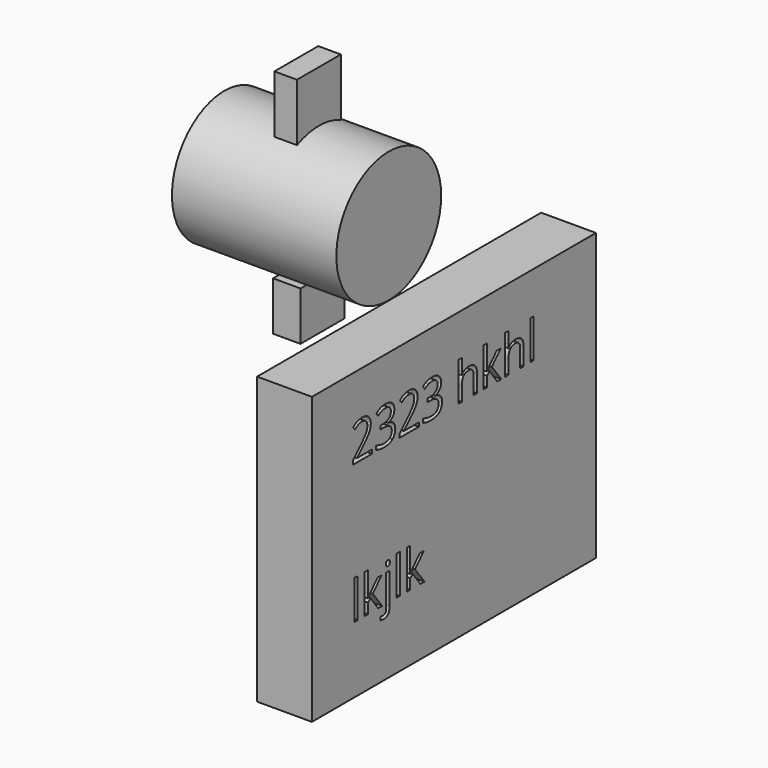
from build123d import *

# Parameters (mm, degrees)
F0_R     = 30.3617666471
F1_DEPTH = 38.1
F2_W     = 12.7535671927
F2_H     = 22.6146032107
F3_DEPTH = 12.7
F4_W     = 10.4644712992
F4_H     = 34.9905658513
F5_DEPTH = 12.7
F6_W     = 164.5638719201
F6_H     = 132.6431203634
F6_W_2   = 1.9235427446
F6_H_2   = 18.0234843295
F7_DEPTH = 25.4


with BuildPart() as f1:
    # F0 (on Right) → F1 (new body, symmetric)
    with BuildSketch(Plane.YZ):
        Circle(F0_R)
    extrude(amount=F1_DEPTH, both=True)

    # F2 (on Front) → F3 (join, symmetric)
    with BuildSketch(Plane.XZ):
        with Locations((0.9810503107, -41.6690682524)):
            Rectangle(F2_W, F2_H)
    extrude(amount=F3_DEPTH, both=True)

    # F4 (on Front) → F5 (join, symmetric)
    with BuildSketch(Plane.XZ):
        with Locations((0.4905241076, 36.7891443893)):
            Rectangle(F4_W, F4_H)
    extrude(amount=F5_DEPTH, both=True)


with BuildPart() as f7:
    # F6 (on face) → F7 (new body)
    with BuildSketch(Plane.YZ.offset(38.1)):
        with Locations((6.0101114213, -96.8088572845)):
            Rectangle(F6_W, F6_H)
        with Locations((-50.736682856, -123.3850151864)):
            Rectangle(F6_W_2, F6_H_2, mode=Mode.SUBTRACT)
        with BuildLine():
            Line((-43.88938956, -125.899704497), (-43.7967333584, -125.899704497))
            add(Edge.make_bspline(
                [(-43.7967333584, -125.899704497), (-43.300096118, -125.191811117), (-42.2808779007, -124.0465804656)],
                knots=[0, 0, 0, 1, 1, 1], degree=2))
            Line((-42.2808779007, -124.0465804656), (-38.1817675432, -119.702857736))
            Line((-38.1817675432, -119.702857736), (-35.8987187365, -119.702857736))
            Line((-35.8987187365, -119.702857736), (-41.0429910477, -125.1102736596))
            Line((-41.0429910477, -125.1102736596), (-35.5392126744, -132.3967573511))
            Line((-35.5392126744, -132.3967573511), (-37.8667364579, -132.3967573511))
            Line((-37.8667364579, -132.3967573511), (-42.3512966139, -126.3963417374))
            Line((-42.3512966139, -126.3963417374), (-43.7967333584, -127.6490535827))
            Line((-43.7967333584, -127.6490535827), (-43.7967333584, -132.3967573511))
            Line((-43.7967333584, -132.3967573511), (-45.6980386146, -132.3967573511))
            Line((-45.6980386146, -132.3967573511), (-45.6980386146, -114.3732730216))
            Line((-45.6980386146, -114.3732730216), (-43.7967333584, -114.3732730216))
            Line((-43.7967333584, -114.3732730216), (-43.7967333584, -123.9316867756))
            add(Edge.make_bspline(
                [(-43.7967333584, -123.9316867756), (-43.7967333584, -124.5654551944), (-43.88938956, -125.899704497)],
                knots=[0, 0, 0, 1, 1, 1], degree=2))
        make_face(mode=Mode.SUBTRACT)
        with BuildLine():
            add(Edge.make_bspline(
                [(-31.325208627, -134.3425375841), (-31.325208627, -138.0969668718), (-34.7905505657, -138.0969668718)],
                knots=[0, 0, 0, 1, 1, 1], degree=2))
            add(Edge.make_bspline(
                [(-34.7905505657, -138.0969668718), (-35.8913062404, -138.0969668718), (-36.5732558839, -137.8041732748)],
                knots=[0, 0, 0, 1, 1, 1], degree=2))
            Line((-36.5732558839, -137.8041732748), (-36.5732558839, -136.2438428403))
            add(Edge.make_bspline(
                [(-36.5732558839, -136.2438428403), (-35.7727063024, -136.4736302202), (-34.9981004572, -136.4736302202)],
                knots=[0, 0, 0, 1, 1, 1], degree=2))
            add(Edge.make_bspline(
                [(-34.9981004572, -136.4736302202), (-34.0937759299, -136.4736302202), (-33.6712636508, -135.9806992279)],
                knots=[0, 0, 0, 1, 1, 1], degree=2))
            add(Edge.make_bspline(
                [(-33.6712636508, -135.9806992279), (-33.2487513716, -135.4877682355), (-33.2487513716, -134.4833750105)],
                knots=[0, 0, 0, 1, 1, 1], degree=2))
            Line((-33.2487513716, -134.4833750105), (-33.2487513716, -119.702857736))
            Line((-33.2487513716, -119.702857736), (-31.325208627, -119.702857736))
            Line((-31.325208627, -119.702857736), (-31.325208627, -134.3425375841))
        make_face(mode=Mode.SUBTRACT)
        with Locations((-26.2865643856, -123.3850151864)):
            Rectangle(F6_W_2, F6_H_2, mode=Mode.SUBTRACT)
        with BuildLine():
            Line((-19.4392710895, -125.899704497), (-19.3466148879, -125.899704497))
            add(Edge.make_bspline(
                [(-19.3466148879, -125.899704497), (-18.8499776475, -125.191811117), (-17.8307594302, -124.0465804656)],
                knots=[0, 0, 0, 1, 1, 1], degree=2))
            Line((-17.8307594302, -124.0465804656), (-13.7316490728, -119.702857736))
            Line((-13.7316490728, -119.702857736), (-11.4486002661, -119.702857736))
            Line((-11.4486002661, -119.702857736), (-16.5928725773, -125.1102736596))
            Line((-16.5928725773, -125.1102736596), (-11.089094204, -132.3967573511))
            Line((-11.089094204, -132.3967573511), (-13.4166179874, -132.3967573511))
            Line((-13.4166179874, -132.3967573511), (-17.9011781434, -126.3963417374))
            Line((-17.9011781434, -126.3963417374), (-19.3466148879, -127.6490535827))
            Line((-19.3466148879, -127.6490535827), (-19.3466148879, -132.3967573511))
            Line((-19.3466148879, -132.3967573511), (-21.2479201442, -132.3967573511))
            Line((-21.2479201442, -132.3967573511), (-21.2479201442, -114.3732730216))
            Line((-21.2479201442, -114.3732730216), (-19.3466148879, -114.3732730216))
            Line((-19.3466148879, -114.3732730216), (-19.3466148879, -123.9316867756))
            add(Edge.make_bspline(
                [(-19.3466148879, -123.9316867756), (-19.3466148879, -124.5654551944), (-19.4392710895, -125.899704497)],
                knots=[0, 0, 0, 1, 1, 1], degree=2))
        make_face(mode=Mode.SUBTRACT)
        with BuildLine():
            add(Edge.make_bspline(
                [(-33.0875295809, -117.2307902781), (-33.4118262864, -116.9120529447), (-33.4118262864, -116.2634595337)],
                knots=[0, 0, 0, 1, 1, 1], degree=2))
            add(Edge.make_bspline(
                [(-33.4118262864, -116.2634595337), (-33.4118262864, -115.6037473785), (-33.0875295809, -115.2961287893)],
                knots=[0, 0, 0, 1, 1, 1], degree=2))
            add(Edge.make_bspline(
                [(-33.0875295809, -115.2961287893), (-32.7632328754, -114.9885102), (-32.2740081311, -114.9885102)],
                knots=[0, 0, 0, 1, 1, 1], degree=2))
            add(Edge.make_bspline(
                [(-32.2740081311, -114.9885102), (-31.8107271232, -114.9885102), (-31.4753116735, -115.3016881614)],
                knots=[0, 0, 0, 1, 1, 1], degree=2))
            add(Edge.make_bspline(
                [(-31.4753116735, -115.3016881614), (-31.1398962238, -115.6148661227), (-31.1398962238, -116.2634595337)],
                knots=[0, 0, 0, 1, 1, 1], degree=2))
            add(Edge.make_bspline(
                [(-31.1398962238, -116.2634595337), (-31.1398962238, -116.9120529447), (-31.4753116735, -117.2307902781)],
                knots=[0, 0, 0, 1, 1, 1], degree=2))
            add(Edge.make_bspline(
                [(-31.4753116735, -117.2307902781), (-31.8107271232, -117.5495276115), (-32.2740081311, -117.5495276115)],
                knots=[0, 0, 0, 1, 1, 1], degree=2))
            add(Edge.make_bspline(
                [(-32.2740081311, -117.5495276115), (-32.7632328754, -117.5495276115), (-33.0875295809, -117.2307902781)],
                knots=[0, 0, 0, 1, 1, 1], degree=2))
        make_face(mode=Mode.SUBTRACT)
        with BuildLine():
            Line((-41.4469720866, -66.0956857553), (-41.4469720866, -67.8783910735))
            Line((-41.4469720866, -67.8783910735), (-52.5768350192, -67.8783910735))
            Line((-52.5768350192, -67.8783910735), (-52.5768350192, -66.2216981894))
            Line((-52.5768350192, -66.2216981894), (-48.1182185996, -61.7408442815))
            add(Edge.make_bspline(
                [(-48.1182185996, -61.7408442815), (-46.0797821651, -59.6764641105), (-45.4311887541, -58.7962301955)],
                knots=[0, 0, 0, 1, 1, 1], degree=2))
            add(Edge.make_bspline(
                [(-45.4311887541, -58.7962301955), (-44.7825953431, -57.9159962806), (-44.4582986376, -57.0820904665)],
                knots=[0, 0, 0, 1, 1, 1], degree=2))
            add(Edge.make_bspline(
                [(-44.4582986376, -57.0820904665), (-44.1340019321, -56.2481846524), (-44.1340019321, -55.2882664041)],
                knots=[0, 0, 0, 1, 1, 1], degree=2))
            add(Edge.make_bspline(
                [(-44.1340019321, -55.2882664041), (-44.1340019321, -53.9317796131), (-44.9567890021, -53.1386425276)],
                knots=[0, 0, 0, 1, 1, 1], degree=2))
            add(Edge.make_bspline(
                [(-44.9567890021, -53.1386425276), (-45.779576072, -52.3455054422), (-47.2398378088, -52.3455054422)],
                knots=[0, 0, 0, 1, 1, 1], degree=2))
            add(Edge.make_bspline(
                [(-47.2398378088, -52.3455054422), (-48.2924122586, -52.3455054422), (-49.2375055146, -52.6938927601)],
                knots=[0, 0, 0, 1, 1, 1], degree=2))
            add(Edge.make_bspline(
                [(-49.2375055146, -52.6938927601), (-50.1825987706, -53.042280078), (-51.3389481662, -53.9577233495)],
                knots=[0, 0, 0, 1, 1, 1], degree=2))
            Line((-51.3389481662, -53.9577233495), (-52.3581663835, -52.6494177833))
            add(Edge.make_bspline(
                [(-52.3581663835, -52.6494177833), (-50.0195238559, -50.7036375504), (-47.2620752971, -50.7036375504)],
                knots=[0, 0, 0, 1, 1, 1], degree=2))
            add(Edge.make_bspline(
                [(-47.2620752971, -50.7036375504), (-44.8752515447, -50.7036375504), (-43.5206178777, -51.9248462871)],
                knots=[0, 0, 0, 1, 1, 1], degree=2))
            add(Edge.make_bspline(
                [(-43.5206178777, -51.9248462871), (-42.1659842107, -53.1460550238), (-42.1659842107, -55.2067289467)],
                knots=[0, 0, 0, 1, 1, 1], degree=2))
            add(Edge.make_bspline(
                [(-42.1659842107, -55.2067289467), (-42.1659842107, -56.818946854), (-43.0703087381, -58.3941022807)],
                knots=[0, 0, 0, 1, 1, 1], degree=2))
            add(Edge.make_bspline(
                [(-43.0703087381, -58.3941022807), (-43.9746332654, -59.9692577074), (-46.4504069714, -62.3783189483)],
                knots=[0, 0, 0, 1, 1, 1], degree=2))
            Line((-46.4504069714, -62.3783189483), (-50.1566550342, -66.0030295537))
            Line((-50.1566550342, -66.0030295537), (-50.1566550342, -66.0956857553))
            Line((-50.1566550342, -66.0956857553), (-41.4469720866, -66.0956857553))
        make_face(mode=Mode.SUBTRACT)
        with BuildLine():
            add(Edge.make_bspline(
                [(-29.8908906267, -51.8321900855), (-28.5232850915, -52.9607426206), (-28.5232850915, -54.928760342)],
                knots=[0, 0, 0, 1, 1, 1], degree=2))
            add(Edge.make_bspline(
                [(-28.5232850915, -54.928760342), (-28.5232850915, -56.5520969935), (-29.4331689909, -57.582433955)],
                knots=[0, 0, 0, 1, 1, 1], degree=2))
            add(Edge.make_bspline(
                [(-29.4331689909, -57.582433955), (-30.3430528903, -58.6127709164), (-32.0108645186, -58.9611582343)],
                knots=[0, 0, 0, 1, 1, 1], degree=2))
            Line((-32.0108645186, -58.9611582343), (-32.0108645186, -59.0538144359))
            add(Edge.make_bspline(
                [(-32.0108645186, -59.0538144359), (-29.9724280841, -59.3058393042), (-28.9884192234, -60.3491481339)],
                knots=[0, 0, 0, 1, 1, 1], degree=2))
            add(Edge.make_bspline(
                [(-28.9884192234, -60.3491481339), (-28.0044103627, -61.3924569636), (-28.0044103627, -63.0825060802)],
                knots=[0, 0, 0, 1, 1, 1], degree=2))
            add(Edge.make_bspline(
                [(-28.0044103627, -63.0825060802), (-28.0044103627, -65.5026860652), (-29.6833407352, -66.8072853833)],
                knots=[0, 0, 0, 1, 1, 1], degree=2))
            add(Edge.make_bspline(
                [(-29.6833407352, -66.8072853833), (-31.3622711076, -68.1118847015), (-34.453281992, -68.1118847015)],
                knots=[0, 0, 0, 1, 1, 1], degree=2))
            add(Edge.make_bspline(
                [(-34.453281992, -68.1118847015), (-35.7986500388, -68.1118847015), (-36.9160838298, -67.908041058)],
                knots=[0, 0, 0, 1, 1, 1], degree=2))
            add(Edge.make_bspline(
                [(-36.9160838298, -67.908041058), (-38.0335176207, -67.7041974145), (-39.0860920705, -67.1964414299)],
                knots=[0, 0, 0, 1, 1, 1], degree=2))
            Line((-39.0860920705, -67.1964414299), (-39.0860920705, -65.3655548869))
            add(Edge.make_bspline(
                [(-39.0860920705, -65.3655548869), (-37.9853363959, -65.9103733521), (-36.7400370468, -66.1939013289)],
                knots=[0, 0, 0, 1, 1, 1], degree=2))
            add(Edge.make_bspline(
                [(-36.7400370468, -66.1939013289), (-35.4947376977, -66.4774293057), (-34.3828632788, -66.4774293057)],
                knots=[0, 0, 0, 1, 1, 1], degree=2))
            add(Edge.make_bspline(
                [(-34.3828632788, -66.4774293057), (-29.9946655724, -66.4774293057), (-29.9946655724, -63.0380311034)],
                knots=[0, 0, 0, 1, 1, 1], degree=2))
            add(Edge.make_bspline(
                [(-29.9946655724, -63.0380311034), (-29.9946655724, -59.9544327152), (-34.8350255425, -59.9544327152)],
                knots=[0, 0, 0, 1, 1, 1], degree=2))
            Line((-34.8350255425, -59.9544327152), (-36.5028371708, -59.9544327152))
            Line((-36.5028371708, -59.9544327152), (-36.5028371708, -58.3014460792))
            Line((-36.5028371708, -58.3014460792), (-34.8127880541, -58.3014460792))
            add(Edge.make_bspline(
                [(-34.8127880541, -58.3014460792), (-32.8336515886, -58.3014460792), (-31.6754490689, -57.4267715363)],
                knots=[0, 0, 0, 1, 1, 1], degree=2))
            add(Edge.make_bspline(
                [(-31.6754490689, -57.4267715363), (-30.5172465493, -56.5520969935), (-30.5172465493, -54.9991790552)],
                knots=[0, 0, 0, 1, 1, 1], degree=2))
            add(Edge.make_bspline(
                [(-30.5172465493, -54.9991790552), (-30.5172465493, -53.7612922022), (-31.3678304797, -53.0533988222)],
                knots=[0, 0, 0, 1, 1, 1], degree=2))
            add(Edge.make_bspline(
                [(-31.3678304797, -53.0533988222), (-32.2184144101, -52.3455054422), (-33.6786761469, -52.3455054422)],
                knots=[0, 0, 0, 1, 1, 1], degree=2))
            add(Edge.make_bspline(
                [(-33.6786761469, -52.3455054422), (-34.7905505657, -52.3455054422), (-35.7745594264, -52.6475646593)],
                knots=[0, 0, 0, 1, 1, 1], degree=2))
            add(Edge.make_bspline(
                [(-35.7745594264, -52.6475646593), (-36.7585682871, -52.9496238764), (-38.0223988765, -53.7612922022)],
                knots=[0, 0, 0, 1, 1, 1], degree=2))
            Line((-38.0223988765, -53.7612922022), (-38.993435869, -52.4641053802))
            add(Edge.make_bspline(
                [(-38.993435869, -52.4641053802), (-37.9519801633, -51.6413183103), (-36.5917871243, -51.1724779303)],
                knots=[0, 0, 0, 1, 1, 1], degree=2))
            add(Edge.make_bspline(
                [(-36.5917871243, -51.1724779303), (-35.2315940852, -50.7036375504), (-33.7231511236, -50.7036375504)],
                knots=[0, 0, 0, 1, 1, 1], degree=2))
            add(Edge.make_bspline(
                [(-33.7231511236, -50.7036375504), (-31.2584961619, -50.7036375504), (-29.8908906267, -51.8321900855)],
                knots=[0, 0, 0, 1, 1, 1], degree=2))
        make_face(mode=Mode.SUBTRACT)
        with BuildLine():
            Line((-14.3246487628, -66.0956857553), (-14.3246487628, -67.8783910735))
            Line((-14.3246487628, -67.8783910735), (-25.4545116955, -67.8783910735))
            Line((-25.4545116955, -67.8783910735), (-25.4545116955, -66.2216981894))
            Line((-25.4545116955, -66.2216981894), (-20.9958952759, -61.7408442815))
            add(Edge.make_bspline(
                [(-20.9958952759, -61.7408442815), (-18.9574588413, -59.6764641105), (-18.3088654304, -58.7962301955)],
                knots=[0, 0, 0, 1, 1, 1], degree=2))
            add(Edge.make_bspline(
                [(-18.3088654304, -58.7962301955), (-17.6602720194, -57.9159962806), (-17.3359753139, -57.0820904665)],
                knots=[0, 0, 0, 1, 1, 1], degree=2))
            add(Edge.make_bspline(
                [(-17.3359753139, -57.0820904665), (-17.0116786084, -56.2481846524), (-17.0116786084, -55.2882664041)],
                knots=[0, 0, 0, 1, 1, 1], degree=2))
            add(Edge.make_bspline(
                [(-17.0116786084, -55.2882664041), (-17.0116786084, -53.9317796131), (-17.8344656783, -53.1386425276)],
                knots=[0, 0, 0, 1, 1, 1], degree=2))
            add(Edge.make_bspline(
                [(-17.8344656783, -53.1386425276), (-18.6572527483, -52.3455054422), (-20.117514485, -52.3455054422)],
                knots=[0, 0, 0, 1, 1, 1], degree=2))
            add(Edge.make_bspline(
                [(-20.117514485, -52.3455054422), (-21.1700889349, -52.3455054422), (-22.1151821909, -52.6938927601)],
                knots=[0, 0, 0, 1, 1, 1], degree=2))
            add(Edge.make_bspline(
                [(-22.1151821909, -52.6938927601), (-23.0602754469, -53.042280078), (-24.2166248425, -53.9577233495)],
                knots=[0, 0, 0, 1, 1, 1], degree=2))
            Line((-24.2166248425, -53.9577233495), (-25.2358430598, -52.6494177833))
            add(Edge.make_bspline(
                [(-25.2358430598, -52.6494177833), (-22.8972005321, -50.7036375504), (-20.1397519734, -50.7036375504)],
                knots=[0, 0, 0, 1, 1, 1], degree=2))
            add(Edge.make_bspline(
                [(-20.1397519734, -50.7036375504), (-17.7529282209, -50.7036375504), (-16.398294554, -51.9248462871)],
                knots=[0, 0, 0, 1, 1, 1], degree=2))
            add(Edge.make_bspline(
                [(-16.398294554, -51.9248462871), (-15.043660887, -53.1460550238), (-15.043660887, -55.2067289467)],
                knots=[0, 0, 0, 1, 1, 1], degree=2))
            add(Edge.make_bspline(
                [(-15.043660887, -55.2067289467), (-15.043660887, -56.818946854), (-15.9479854143, -58.3941022807)],
                knots=[0, 0, 0, 1, 1, 1], degree=2))
            add(Edge.make_bspline(
                [(-15.9479854143, -58.3941022807), (-16.8523099417, -59.9692577074), (-19.3280836476, -62.3783189483)],
                knots=[0, 0, 0, 1, 1, 1], degree=2))
            Line((-19.3280836476, -62.3783189483), (-23.0343317105, -66.0030295537))
            Line((-23.0343317105, -66.0030295537), (-23.0343317105, -66.0956857553))
            Line((-23.0343317105, -66.0956857553), (-14.3246487628, -66.0956857553))
        make_face(mode=Mode.SUBTRACT)
        with BuildLine():
            add(Edge.make_bspline(
                [(-2.7685673029, -51.8321900855), (-1.4009617677, -52.9607426206), (-1.4009617677, -54.928760342)],
                knots=[0, 0, 0, 1, 1, 1], degree=2))
            add(Edge.make_bspline(
                [(-1.4009617677, -54.928760342), (-1.4009617677, -56.5520969935), (-2.3108456672, -57.582433955)],
                knots=[0, 0, 0, 1, 1, 1], degree=2))
            add(Edge.make_bspline(
                [(-2.3108456672, -57.582433955), (-3.2207295666, -58.6127709164), (-4.8885411949, -58.9611582343)],
                knots=[0, 0, 0, 1, 1, 1], degree=2))
            Line((-4.8885411949, -58.9611582343), (-4.8885411949, -59.0538144359))
            add(Edge.make_bspline(
                [(-4.8885411949, -59.0538144359), (-2.8501047603, -59.3058393042), (-1.8660958996, -60.3491481339)],
                knots=[0, 0, 0, 1, 1, 1], degree=2))
            add(Edge.make_bspline(
                [(-1.8660958996, -60.3491481339), (-0.882087039, -61.3924569636), (-0.882087039, -63.0825060802)],
                knots=[0, 0, 0, 1, 1, 1], degree=2))
            add(Edge.make_bspline(
                [(-0.882087039, -63.0825060802), (-0.882087039, -65.5026860652), (-2.5610174114, -66.8072853833)],
                knots=[0, 0, 0, 1, 1, 1], degree=2))
            add(Edge.make_bspline(
                [(-2.5610174114, -66.8072853833), (-4.2399477839, -68.1118847015), (-7.3309586683, -68.1118847015)],
                knots=[0, 0, 0, 1, 1, 1], degree=2))
            add(Edge.make_bspline(
                [(-7.3309586683, -68.1118847015), (-8.6763267151, -68.1118847015), (-9.793760506, -67.908041058)],
                knots=[0, 0, 0, 1, 1, 1], degree=2))
            add(Edge.make_bspline(
                [(-9.793760506, -67.908041058), (-10.911194297, -67.7041974145), (-11.9637687468, -67.1964414299)],
                knots=[0, 0, 0, 1, 1, 1], degree=2))
            Line((-11.9637687468, -67.1964414299), (-11.9637687468, -65.3655548869))
            add(Edge.make_bspline(
                [(-11.9637687468, -65.3655548869), (-10.8630130721, -65.9103733521), (-9.617713723, -66.1939013289)],
                knots=[0, 0, 0, 1, 1, 1], degree=2))
            add(Edge.make_bspline(
                [(-9.617713723, -66.1939013289), (-8.3724143739, -66.4774293057), (-7.2605399551, -66.4774293057)],
                knots=[0, 0, 0, 1, 1, 1], degree=2))
            add(Edge.make_bspline(
                [(-7.2605399551, -66.4774293057), (-2.8723422487, -66.4774293057), (-2.8723422487, -63.0380311034)],
                knots=[0, 0, 0, 1, 1, 1], degree=2))
            add(Edge.make_bspline(
                [(-2.8723422487, -63.0380311034), (-2.8723422487, -59.9544327152), (-7.7127022187, -59.9544327152)],
                knots=[0, 0, 0, 1, 1, 1], degree=2))
            Line((-7.7127022187, -59.9544327152), (-9.380513847, -59.9544327152))
            Line((-9.380513847, -59.9544327152), (-9.380513847, -58.3014460792))
            Line((-9.380513847, -58.3014460792), (-7.6904647304, -58.3014460792))
            add(Edge.make_bspline(
                [(-7.6904647304, -58.3014460792), (-5.7113282648, -58.3014460792), (-4.5531257452, -57.4267715363)],
                knots=[0, 0, 0, 1, 1, 1], degree=2))
            add(Edge.make_bspline(
                [(-4.5531257452, -57.4267715363), (-3.3949232255, -56.5520969935), (-3.3949232255, -54.9991790552)],
                knots=[0, 0, 0, 1, 1, 1], degree=2))
            add(Edge.make_bspline(
                [(-3.3949232255, -54.9991790552), (-3.3949232255, -53.7612922022), (-4.245507156, -53.0533988222)],
                knots=[0, 0, 0, 1, 1, 1], degree=2))
            add(Edge.make_bspline(
                [(-4.245507156, -53.0533988222), (-5.0960910864, -52.3455054422), (-6.5563528231, -52.3455054422)],
                knots=[0, 0, 0, 1, 1, 1], degree=2))
            add(Edge.make_bspline(
                [(-6.5563528231, -52.3455054422), (-7.668227242, -52.3455054422), (-8.6522361027, -52.6475646593)],
                knots=[0, 0, 0, 1, 1, 1], degree=2))
            add(Edge.make_bspline(
                [(-8.6522361027, -52.6475646593), (-9.6362449633, -52.9496238764), (-10.9000755528, -53.7612922022)],
                knots=[0, 0, 0, 1, 1, 1], degree=2))
            Line((-10.9000755528, -53.7612922022), (-11.8711125452, -52.4641053802))
            add(Edge.make_bspline(
                [(-11.8711125452, -52.4641053802), (-10.8296568396, -51.6413183103), (-9.4694638005, -51.1724779303)],
                knots=[0, 0, 0, 1, 1, 1], degree=2))
            add(Edge.make_bspline(
                [(-9.4694638005, -51.1724779303), (-8.1092707615, -50.7036375504), (-6.6008277999, -50.7036375504)],
                knots=[0, 0, 0, 1, 1, 1], degree=2))
            add(Edge.make_bspline(
                [(-6.6008277999, -50.7036375504), (-4.1361728381, -50.7036375504), (-2.7685673029, -51.8321900855)],
                knots=[0, 0, 0, 1, 1, 1], degree=2))
        make_face(mode=Mode.SUBTRACT)
        with BuildLine():
            Line((19.3206711515, -67.8783910735), (17.3971284069, -67.8783910735))
            Line((17.3971284069, -67.8783910735), (17.3971284069, -59.6653453663))
            add(Edge.make_bspline(
                [(17.3971284069, -59.6653453663), (17.3971284069, -58.116133676), (16.6910881509, -57.350793451)],
                knots=[0, 0, 0, 1, 1, 1], degree=2))
            add(Edge.make_bspline(
                [(16.6910881509, -57.350793451), (15.985047895, -56.5854532261), (14.4766049334, -56.5854532261)],
                knots=[0, 0, 0, 1, 1, 1], degree=2))
            add(Edge.make_bspline(
                [(14.4766049334, -56.5854532261), (12.4752309795, -56.5854532261), (11.5542283359, -57.6750901565)],
                knots=[0, 0, 0, 1, 1, 1], degree=2))
            add(Edge.make_bspline(
                [(11.5542283359, -57.6750901565), (10.6332256922, -58.764727087), (10.6332256922, -61.240500793)],
                knots=[0, 0, 0, 1, 1, 1], degree=2))
            Line((10.6332256922, -61.240500793), (10.6332256922, -67.8783910735))
            Line((10.6332256922, -67.8783910735), (8.7096829476, -67.8783910735))
            Line((8.7096829476, -67.8783910735), (8.7096829476, -49.854906744))
            Line((8.7096829476, -49.854906744), (10.6332256922, -49.854906744))
            Line((10.6332256922, -49.854906744), (10.6332256922, -55.3105038925))
            add(Edge.make_bspline(
                [(10.6332256922, -55.3105038925), (10.6332256922, -56.2963658772), (10.5405694907, -56.9449592882)],
                knots=[0, 0, 0, 1, 1, 1], degree=2))
            Line((10.5405694907, -56.9449592882), (10.6554631806, -56.9449592882))
            add(Edge.make_bspline(
                [(10.6554631806, -56.9449592882), (11.2225191342, -56.0295160166), (12.271387336, -55.5032287917)],
                knots=[0, 0, 0, 1, 1, 1], degree=2))
            add(Edge.make_bspline(
                [(12.271387336, -55.5032287917), (13.3202555378, -54.9769415668), (14.6619173365, -54.9769415668)],
                knots=[0, 0, 0, 1, 1, 1], degree=2))
            add(Edge.make_bspline(
                [(14.6619173365, -54.9769415668), (16.98944112, -54.9769415668), (18.1550561357, -56.0832566136)],
                knots=[0, 0, 0, 1, 1, 1], degree=2))
            add(Edge.make_bspline(
                [(18.1550561357, -56.0832566136), (19.3206711515, -57.1895716603), (19.3206711515, -59.5986329011)],
                knots=[0, 0, 0, 1, 1, 1], degree=2))
            Line((19.3206711515, -59.5986329011), (19.3206711515, -67.8783910735))
        make_face(mode=Mode.SUBTRACT)
        with BuildLine():
            Line((25.0764743931, -61.3813382194), (25.1691305946, -61.3813382194))
            add(Edge.make_bspline(
                [(25.1691305946, -61.3813382194), (25.6657678351, -60.6734448394), (26.6849860523, -59.528214188)],
                knots=[0, 0, 0, 1, 1, 1], degree=2))
            Line((26.6849860523, -59.528214188), (30.7840964098, -55.1844914583))
            Line((30.7840964098, -55.1844914583), (33.0671452165, -55.1844914583))
            Line((33.0671452165, -55.1844914583), (27.9228729053, -60.591907382))
            Line((27.9228729053, -60.591907382), (33.4266512786, -67.8783910735))
            Line((33.4266512786, -67.8783910735), (31.0991274952, -67.8783910735))
            Line((31.0991274952, -67.8783910735), (26.6145673391, -61.8779754598))
            Line((26.6145673391, -61.8779754598), (25.1691305946, -63.130687305))
            Line((25.1691305946, -63.130687305), (25.1691305946, -67.8783910735))
            Line((25.1691305946, -67.8783910735), (23.2678253384, -67.8783910735))
            Line((23.2678253384, -67.8783910735), (23.2678253384, -49.854906744))
            Line((23.2678253384, -49.854906744), (25.1691305946, -49.854906744))
            Line((25.1691305946, -49.854906744), (25.1691305946, -59.413320498))
            add(Edge.make_bspline(
                [(25.1691305946, -59.413320498), (25.1691305946, -60.0470889167), (25.0764743931, -61.3813382194)],
                knots=[0, 0, 0, 1, 1, 1], degree=2))
        make_face(mode=Mode.SUBTRACT)
        with BuildLine():
            Line((46.3281007853, -67.8783910735), (44.4045580407, -67.8783910735))
            Line((44.4045580407, -67.8783910735), (44.4045580407, -59.6653453663))
            add(Edge.make_bspline(
                [(44.4045580407, -59.6653453663), (44.4045580407, -58.116133676), (43.6985177847, -57.350793451)],
                knots=[0, 0, 0, 1, 1, 1], degree=2))
            add(Edge.make_bspline(
                [(43.6985177847, -57.350793451), (42.9924775288, -56.5854532261), (41.4840345672, -56.5854532261)],
                knots=[0, 0, 0, 1, 1, 1], degree=2))
            add(Edge.make_bspline(
                [(41.4840345672, -56.5854532261), (39.4826606133, -56.5854532261), (38.5616579697, -57.6750901565)],
                knots=[0, 0, 0, 1, 1, 1], degree=2))
            add(Edge.make_bspline(
                [(38.5616579697, -57.6750901565), (37.640655326, -58.764727087), (37.640655326, -61.240500793)],
                knots=[0, 0, 0, 1, 1, 1], degree=2))
            Line((37.640655326, -61.240500793), (37.640655326, -67.8783910735))
            Line((37.640655326, -67.8783910735), (35.7171125814, -67.8783910735))
            Line((35.7171125814, -67.8783910735), (35.7171125814, -49.854906744))
            Line((35.7171125814, -49.854906744), (37.640655326, -49.854906744))
            Line((37.640655326, -49.854906744), (37.640655326, -55.3105038925))
            add(Edge.make_bspline(
                [(37.640655326, -55.3105038925), (37.640655326, -56.2963658772), (37.5479991245, -56.9449592882)],
                knots=[0, 0, 0, 1, 1, 1], degree=2))
            Line((37.5479991245, -56.9449592882), (37.6628928144, -56.9449592882))
            add(Edge.make_bspline(
                [(37.6628928144, -56.9449592882), (38.229948768, -56.0295160166), (39.2788169698, -55.5032287917)],
                knots=[0, 0, 0, 1, 1, 1], degree=2))
            add(Edge.make_bspline(
                [(39.2788169698, -55.5032287917), (40.3276851716, -54.9769415668), (41.6693469703, -54.9769415668)],
                knots=[0, 0, 0, 1, 1, 1], degree=2))
            add(Edge.make_bspline(
                [(41.6693469703, -54.9769415668), (43.9968707538, -54.9769415668), (45.1624857695, -56.0832566136)],
                knots=[0, 0, 0, 1, 1, 1], degree=2))
            add(Edge.make_bspline(
                [(45.1624857695, -56.0832566136), (46.3281007853, -57.1895716603), (46.3281007853, -59.5986329011)],
                knots=[0, 0, 0, 1, 1, 1], degree=2))
            Line((46.3281007853, -59.5986329011), (46.3281007853, -67.8783910735))
        make_face(mode=Mode.SUBTRACT)
        with Locations((51.2370263445, -58.8666489087)):
            Rectangle(F6_W_2, F6_H_2, mode=Mode.SUBTRACT)
    extrude(amount=F7_DEPTH)


solid = Compound([f1.part, f7.part])
